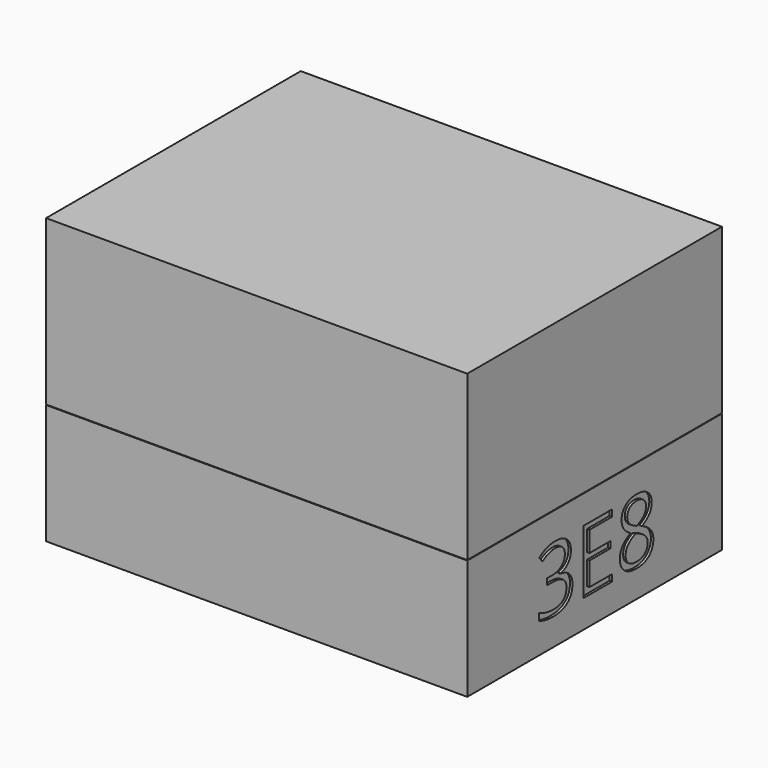
from build123d import *

# Parameters (mm, degrees)
F0_W          = 86
F0_H          = 65
F1_DEPTH      = 2
F2_W          = 86
F2_H          = 65
F2_W_2        = 82
F2_H_2        = 61
F3_DEPTH      = 22.5
F4_W          = 83.4
F4_H          = 62.4
F4_W_2        = 82
F4_H_2        = 61
F5_DEPTH      = 5
F7_W          = 86
F7_H          = 65
F8_DEPTH      = 28.5
F9_W          = 82
F9_H          = 61
F10_DEPTH     = 26.5
F11_W         = 86
F11_H         = 65
F11_W_2       = 84.6
F11_H_2       = 63.6
F12_DEPTH     = 5
F13_TEXT_SIZE = 18.2069765197
F14_DEPTH     = 0.5


# Not quite as in the source:
# - Text() gives the source's letters only with a copy of the font that has no kerning and outlines rounded to 1/6400 em; it was checked with that copy


with BuildPart() as f1:
    # F0 (on Top) → F1 (new body)
    with BuildSketch(Plane.XY):
        Rectangle(F0_W, F0_H)
    extrude(amount=F1_DEPTH)

    # F2 (on face) → F3 (join)
    with BuildSketch(Plane.XY.offset(2)):
        Rectangle(F2_W, F2_H)
        Rectangle(F2_W_2, F2_H_2, mode=Mode.SUBTRACT)
    extrude(amount=F3_DEPTH)

    # F4 (on face) → F5 (join)
    with BuildSketch(Plane.XY.offset(24.5)):
        Rectangle(F4_W, F4_H)
        Rectangle(F4_W_2, F4_H_2, mode=Mode.SUBTRACT)
    extrude(amount=F5_DEPTH)

    # F13 (on face) → F14 (cut)
    with BuildSketch(Plane.YZ.offset(43)):
        with Locations((-15.0008417482, 5.6954884529)):
            Text('3E8', F13_TEXT_SIZE, font='Open Sans', text_align=(TextAlign.LEFT, TextAlign.BOTTOM))
    extrude(amount=-F14_DEPTH, mode=Mode.SUBTRACT)


with BuildPart() as f8:
    # F7 (on offset) → F8 (new body)
    with BuildSketch(Plane.XY.offset(29.6)):
        Rectangle(F7_W, F7_H)
    extrude(amount=F8_DEPTH)

    # F9 (on face) → F10 (cut)
    with BuildSketch(Plane(origin=(0, 0, 29.6), x_dir=(1, 0, 0), z_dir=(0, 0, -1))):
        Rectangle(F9_W, F9_H)
    extrude(amount=-F10_DEPTH, mode=Mode.SUBTRACT)

    # F11 (on face) → F12 (join)
    with BuildSketch(Plane(origin=(0, 0, 29.6), x_dir=(1, 0, 0), z_dir=(0, 0, -1))):
        Rectangle(F11_W, F11_H)
        Rectangle(F11_W_2, F11_H_2, mode=Mode.SUBTRACT)
    extrude(amount=F12_DEPTH)


solid = Compound([f1.part, f8.part])
